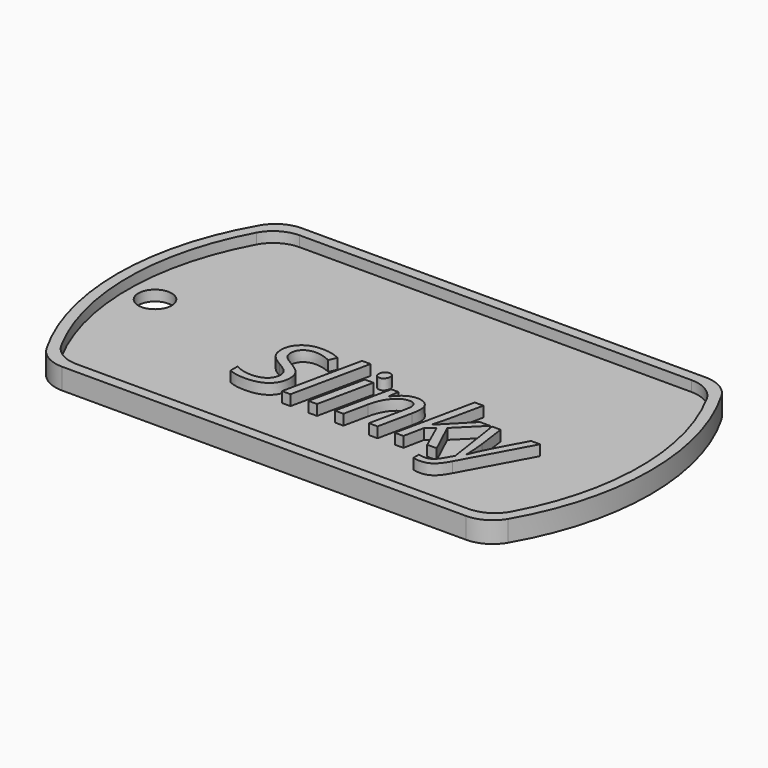
from build123d import *

# Parameters (mm, degrees)
F1_DEPTH      = 1
F3_DEPTH      = 1
F4_R          = 1.5875
F5_DEPTH      = 1
F8_TEXT_SIZE  = 6.9561815407
F7_TEXT_SIZE  = 6.9561821874
F6_TEXT_SIZE  = 6.9561815407
F9_DEPTH      = 1
F10_TEXT_SIZE = 9.9073823852
F11_DEPTH     = 1


# Not quite as in the source:
# - Text() gives the source's letters only with a copy of the font that has no kerning and outlines rounded to 1/6400 em; it was checked with that copy


with BuildPart() as f1:
    # F0 (on Top) → F1 (new body)
    with BuildSketch(Plane.XY):
        with BuildLine():
            ThreePointArc((-19.2474145991, 14.2875), (-20.8349145991, 13.862130657), (-21.9970452561, 12.7))
            ThreePointArc((-21.9970452561, 12.7), (-25.4, 0), (-21.9970452561, -12.7))
            ThreePointArc((-21.9970452561, -12.7), (-20.8349145991, -13.862130657), (-19.2474145991, -14.2875))
            Line((-19.2474145991, -14.2875), (19.2474145991, -14.2875))
            ThreePointArc((19.2474145991, -14.2875), (20.8349145991, -13.862130657), (21.9970452561, -12.7))
            ThreePointArc((21.9970452561, -12.7), (25.4, 0), (21.9970452561, 12.7))
            ThreePointArc((21.9970452561, 12.7), (20.8349145991, 13.862130657), (19.2474145991, 14.2875))
            Line((19.2474145991, 14.2875), (-19.2474145991, 14.2875))
        make_face()
    extrude(amount=F1_DEPTH)

    # F2 (on face) → F3 (join)
    with BuildSketch(Plane.XY.offset(1)):
        with BuildLine():
            Line((19.2474145991, 14.2875), (-19.2474145991, 14.2875))
            ThreePointArc((-19.2474145991, 14.2875), (-20.8349145991, 13.862130657), (-21.9970452561, 12.7))
            ThreePointArc((-21.9970452561, 12.7), (-25.4, 0), (-21.9970452561, -12.7))
            ThreePointArc((-21.9970452561, -12.7), (-20.8349145991, -13.862130657), (-19.2474145991, -14.2875))
            Line((-19.2474145991, -14.2875), (19.2474145991, -14.2875))
            ThreePointArc((19.2474145991, -14.2875), (20.8349145991, -13.862130657), (21.9970452561, -12.7))
            ThreePointArc((21.9970452561, -12.7), (25.4, 0), (21.9970452561, 12.7))
            ThreePointArc((21.9970452561, 12.7), (20.8349145991, 13.862130657), (19.2474145991, 14.2875))
        make_face()
        with BuildLine():
            ThreePointArc((-21.4526124879, 11.6252061249), (-20.2856017842, 12.8404540819), (-18.6611352482, 13.2875))
            Line((-18.6611352482, 13.2875), (18.6611352482, 13.2875))
            ThreePointArc((18.6611352482, 13.2875), (20.2856017842, 12.8404540819), (21.4526124879, 11.6252061249))
            ThreePointArc((21.4526124879, 11.6252061249), (24.4, 0), (21.4526124879, -11.6252061249))
            ThreePointArc((21.4526124879, -11.6252061249), (20.2856017842, -12.8404540819), (18.6611352482, -13.2875))
            Line((18.6611352482, -13.2875), (-18.6611352482, -13.2875))
            ThreePointArc((-18.6611352482, -13.2875), (-20.2856017842, -12.8404540819), (-21.4526124879, -11.6252061249))
            ThreePointArc((-21.4526124879, -11.6252061249), (-24.4, 0), (-21.4526124879, 11.6252061249))
        make_face(mode=Mode.SUBTRACT)
    extrude(amount=F3_DEPTH)

    # F4 (on face) → F5 (cut)
    with BuildSketch(Plane.XY.offset(1)):
        with Locations((-21.821282804, 0)):
            Circle(F4_R)
    extrude(amount=-F5_DEPTH, mode=Mode.SUBTRACT)

    # F8 (on face) + F7 (on face) + F6 (on face) → F9 (join)
    with BuildSketch(Plane(origin=(0, 0, 0), x_dir=(1, 0, 0), z_dir=(0, 0, -1))):
        with Locations((-18.9069006592, 0)):
            Text('M & D BFFL', F8_TEXT_SIZE, font='Open Sans', text_align=(TextAlign.LEFT, TextAlign.BOTTOM))
    with BuildSketch(Plane.XY.offset(1)):
        with Locations((-6.6361962818, -12.7715496346)):
            Text('Adams', F7_TEXT_SIZE, font='Open Sans', font_style=FontStyle.ITALIC, text_align=(TextAlign.LEFT, TextAlign.BOTTOM))
    with BuildSketch(Plane.XY.offset(1)):
        with Locations((-6.385773886, -5.0084507093)):
            Text('Drew', F6_TEXT_SIZE, font='Open Sans', font_style=FontStyle.ITALIC, text_align=(TextAlign.LEFT, TextAlign.BOTTOM))
    extrude(amount=F9_DEPTH, dir=(0, 0, -1))

    # F10 (on face) → F11 (join)
    with BuildSketch(Plane.XY.offset(1)):
        with Locations((-9.2654237524, -7.1333153173)):
            Text('Slinky', F10_TEXT_SIZE, font='Open Sans', font_style=FontStyle.ITALIC, text_align=(TextAlign.LEFT, TextAlign.BOTTOM))
    extrude(amount=F11_DEPTH)


solid = f1.part
